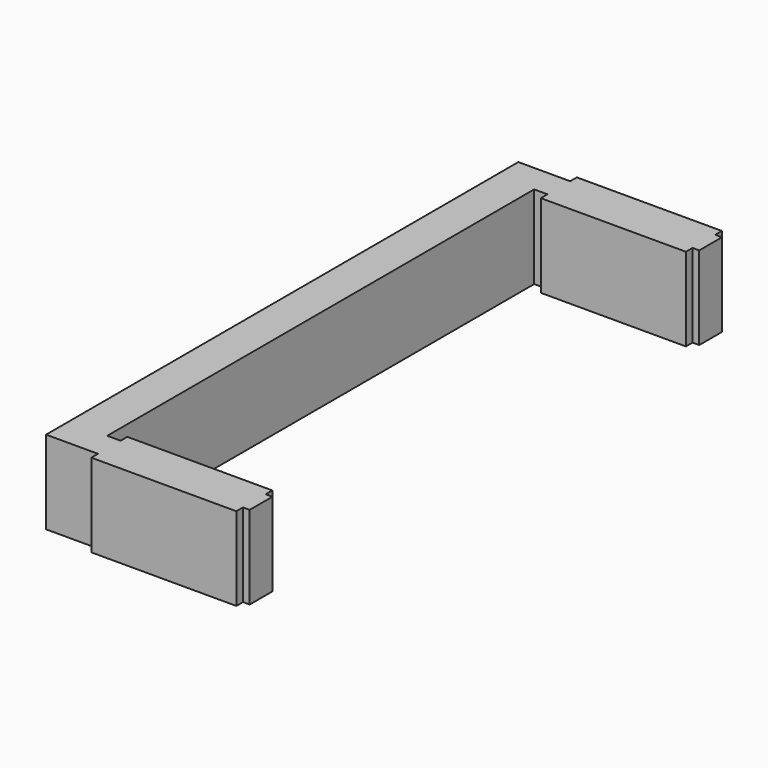
from build123d import *

# Parameters (mm, degrees)
F0_W     = 22.098
F0_H     = 4.318
F0_W_2   = 2.032
F0_H_2   = 1.27
F0_W_3   = 1.016
F1_DEPTH = 12.7
F2_DEPTH = 12.7


# Not quite as in the source:
# - a feature names something its author has since deleted; it is built from what else it names


with BuildPart() as f1:
    # F0 (on Top) → F1 (new body)
    with BuildSketch(Plane.XY):
        with Locations((-31.8938936177, -48.641)):
            Rectangle(F0_W, F0_H)
        with Locations((-43.9588936177, -48.641)):
            Rectangle(F0_W_2, F0_H)
        with Locations((-31.8938936177, -51.435)):
            Rectangle(F0_W, F0_H_2)
        with Locations((-31.8938936177, -45.847)):
            Rectangle(F0_W, F0_H_2)
        with Locations((-20.3368936177, -48.641)):
            Rectangle(F0_W_3, F0_H)
        Polygon((-50.8410629748, -50.8), (-44.9748936177, -50.8), (-44.9748936177, -46.482), (-44.9748936177, 34.798), (-44.9748936177, 39.116), (-50.8410629748, 39.116), align=None)
    extrude(amount=F1_DEPTH)

    # F0 (on Top) → F2 (join)
    with BuildSketch(Plane.XY):
        with Locations((-31.8938936177, 36.957)):
            Rectangle(F0_W, F0_H)
        with Locations((-43.9588936177, 36.957)):
            Rectangle(F0_W_2, F0_H)
        with Locations((-31.8938936177, 34.163)):
            Rectangle(F0_W, F0_H_2)
        with Locations((-31.8938936177, 39.751)):
            Rectangle(F0_W, F0_H_2)
        with Locations((-20.3368936177, 36.957)):
            Rectangle(F0_W_3, F0_H)
    extrude(amount=F2_DEPTH)


solid = f1.part
